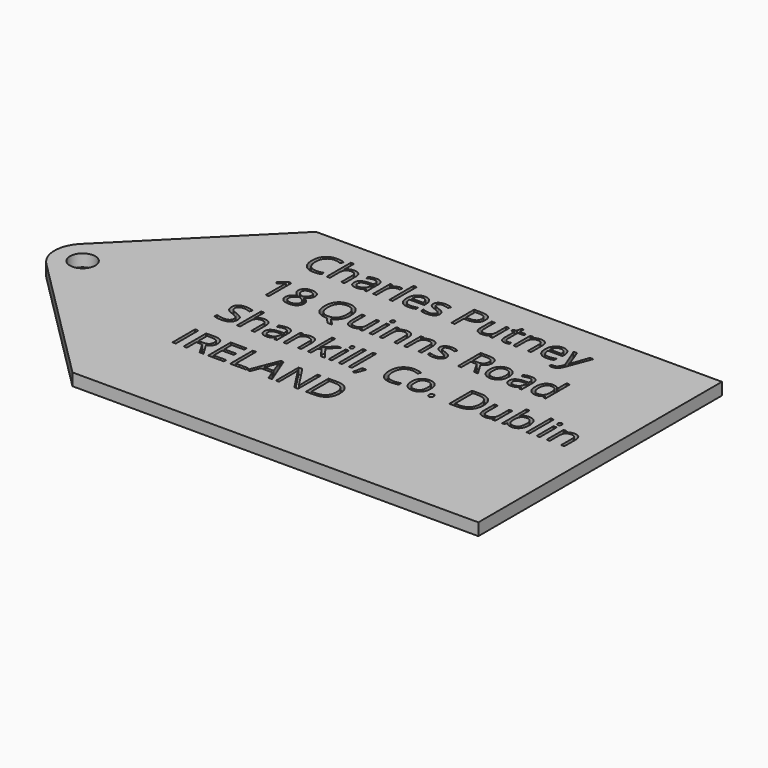
from build123d import *

# Parameters (mm, degrees)
F0_R         = 2.5
F0_W         = 80
F0_H         = 60
F1_DEPTH     = 2.4
F2_TEXT_SIZE = 7.8283357797
F3_DEPTH     = 1.2


# Not quite as in the source:
# - Text() gives the source's letters only with a copy of the font that has no kerning and outlines rounded to 1/6400 em; it was checked with that copy


with BuildPart() as f1:
    # F0 (on Top) → F1 (new body)
    with BuildSketch(Plane.XY):
        with BuildLine():
            Line((-23.865801543, -30), (-23.865801543, 30))
            Line((-23.865801543, 30), (-49.6231608559, 4.2426406871))
            ThreePointArc((-49.6231608559, 4.2426406871), (-51.3805201688, 0), (-49.6231608559, -4.2426406871))
            Line((-49.6231608559, -4.2426406871), (-23.865801543, -30))
        make_face()
        with Locations((-45.865801543, 0)):
            Circle(F0_R, mode=Mode.SUBTRACT)
        with Locations((16.134198457, 0)):
            Rectangle(F0_W, F0_H)
    extrude(amount=F1_DEPTH)

    # F2 (on face) → F3 (cut)
    with BuildSketch(Plane.XY.offset(2.4)):
        with Locations((-18.865801543, 19.3635982386)):
            Text('Charles Putney', F2_TEXT_SIZE, font='Open Sans', text_align=(TextAlign.LEFT, TextAlign.BOTTOM))
        with Locations((-18.865801543, 8.7170615782)):
            Text('18 Quinns Road', F2_TEXT_SIZE, font='Open Sans', text_align=(TextAlign.LEFT, TextAlign.BOTTOM))
        with Locations((-18.865801543, -1.9294750821)):
            Text('Shankill, Co. Dublin', F2_TEXT_SIZE, font='Open Sans', text_align=(TextAlign.LEFT, TextAlign.BOTTOM))
        with Locations((-18.865801543, -12.5760117425)):
            Text('IRELAND', F2_TEXT_SIZE, font='Open Sans', text_align=(TextAlign.LEFT, TextAlign.BOTTOM))
    extrude(amount=-F3_DEPTH, mode=Mode.SUBTRACT)


solid = f1.part
